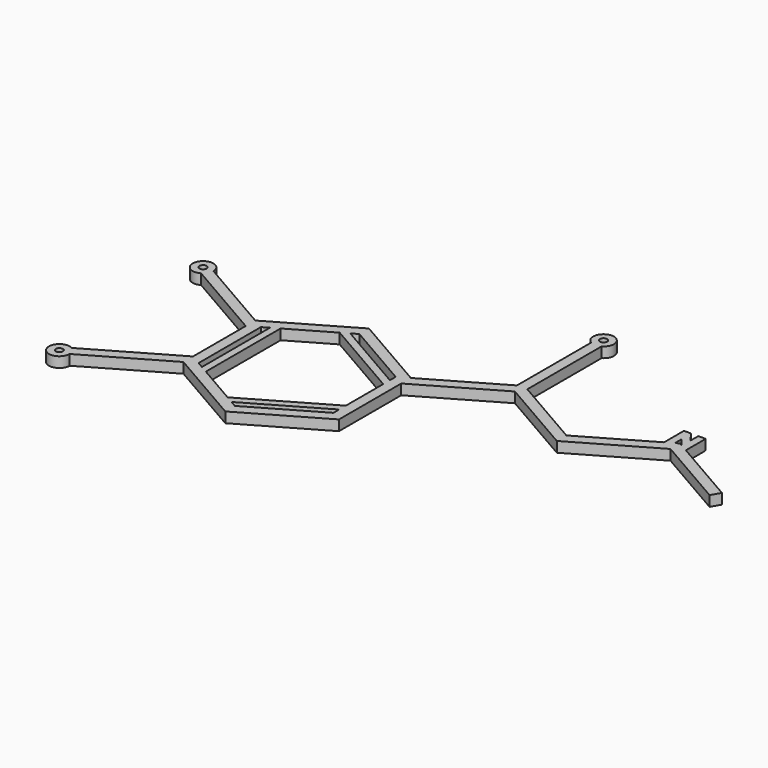
from build123d import *

# Parameters (mm, degrees)
F0_R     = 0.4318
F0_R_2   = 0.4445
F1_DEPTH = 1.27
F3_DEPTH = 1.27


# Not quite as in the source:
# - ends of sketch curves that miss each other by under 0.0002 mm in the source are joined


with BuildPart() as f1:
    # F0 (on Top) → F1 (new body)
    with BuildSketch(Plane.XY):
        with BuildLine():
            Line((9.5249989071, 5.499263207), (-2.1858e-06, 10.9985226281))
            Line((-2.1858e-06, 10.9985226281), (-9.5250010929, 5.499259421))
            Line((-9.5250010929, 5.499259421), (-19.0459112442, 10.9961569369))
            ThreePointArc((-19.0459112442, 10.9961569369), (-21.4157534444, 11.6311591353), (-19.6809068475, 9.8963021357))
            Line((-19.6809068475, 9.8963021357), (-9.5250008015, 4.0327897373))
            Line((-9.5250008015, 4.0327897373), (-9.5249991985, -4.0327941963))
            Line((-9.5249991985, -4.0327941963), (-19.6850080876, -9.8986699867))
            ThreePointArc((-19.6850080876, -9.8986699867), (-21.4198613847, -11.6335212151), (-19.0500087433, -10.9985226281))
            Line((-19.0500087433, -10.9985226281), (-9.5249989071, -5.499263207))
            Line((-9.5249989071, -5.499263207), (2.1858e-06, -10.9985226281))
            Line((2.1858e-06, -10.9985226281), (9.5250010929, -5.499259421))
            Line((9.5250010929, -5.499259421), (9.5249991985, 4.0327941963))
            Line((9.5249991985, 4.0327941963), (19.0500087433, 9.5320534491))
            Line((19.0500087433, 9.5320534491), (28.5750185796, 4.0327940281))
            Line((28.5750185796, 4.0327940281), (38.1000284158, 9.5320534491))
            Line((38.1000284158, 9.5320534491), (46.9900389078, 4.3994105656))
            Line((46.9900389078, 4.3994105656), (47.625038252, 5.499263207))
            Line((47.625038252, 5.499263207), (39.3991596309, 10.2484699041))
            Line((39.3991596309, 10.2484699041), (39.3991596309, 10.224751758))
            Line((39.3991596309, 10.224751758), (38.673771624, 10.6672722885))
            Line((38.673771624, 10.6672722885), (38.1000284158, 10.9985226281))
            Line((38.1000284158, 10.9985226281), (37.6488161101, 10.7380154406))
            Line((37.6488161101, 10.7380154406), (37.6488161101, 10.731614756))
            Line((37.6488161101, 10.731614756), (36.7598161101, 10.224751758))
            Line((36.7598161101, 10.224751758), (28.5750185796, 5.499263207))
            Line((28.5750185796, 5.499263207), (19.6850087433, 10.6319053096))
            Line((19.6850087433, 10.6319053096), (19.6850087433, 10.9985226281))
            Line((19.6850087433, 10.9985226281), (19.6850087433, 21.9970528281))
            ThreePointArc((19.6850087433, 21.9970528281), (19.0500083949, 24.3669048897), (18.4150080465, 21.9970528281))
            Line((18.4150080465, 21.9970528281), (18.4150080465, 10.9985226281))
            Line((18.4150080465, 10.9985226281), (18.4150080465, 10.6319053096))
            Line((18.4150080465, 10.6319053096), (9.5249989071, 5.499263207))
        make_face()
        with Locations((-20.3200087433, -10.9985218709)):
            Circle(F0_R, mode=Mode.SUBTRACT)
        Polygon((8.2550007723, -3.8861430213), (8.2550009472, -4.7660248316), (1.8944e-06, -9.5320529443), (-0.761998193, -9.0921121906), align=None, mode=Mode.SUBTRACT)
        Polygon((-8.255, -1.6406e-06), (-8.2550009472, 4.7660248316), (-7.493, 5.2059664855), (-7.493, -1.6406e-06), (-7.493, -5.2059682691), (-8.2549990528, -4.7660281127), align=None, mode=Mode.SUBTRACT)
        Polygon((-6.604, -5.499263207), (-6.604, 5.7192311104), (-1.6510017049, 8.5788473218), (8.2549994317, 2.8596175239), (8.2550005683, -2.8596142427), (-1.6509982951, -8.578847978), (-6.604, -5.7192324228), align=None, mode=Mode.SUBTRACT)
        with Locations((-20.3159024508, 10.9961569369)):
            Circle(F0_R_2, mode=Mode.SUBTRACT)
        Polygon((-1.8944e-06, 9.5320529443), (8.2549990528, 4.7660281127), (8.2549992277, 3.8861463025), (-0.762001807, 9.0921118878), align=None, mode=Mode.SUBTRACT)
        with Locations((19.0500083949, 23.0969048897)):
            Circle(F0_R_2, mode=Mode.SUBTRACT)
        Polygon((36.7598161101, 10.731614756), (36.7598161101, 10.224751758), (37.6488161101, 10.7380154406), (37.6488161101, 11.8624546668), (38.5683002365, 10.731614756), (38.673771624, 10.6672722885), (39.3991596309, 10.2484699041), (39.3991596309, 10.731614756), (39.3991596309, 13.271614756), (38.5101596309, 13.271614756), (38.5101596309, 12.0436610678), (37.6488161101, 13.271614756), (36.7598161101, 13.271614756), align=None)
        Polygon((37.6488161101, 10.7380154406), (36.7598161101, 10.224751758), (37.6488161101, 10.731614756), align=None)
        Polygon((39.3991596309, 10.2484699041), (38.673771624, 10.6672722885), (39.3991596309, 10.224751758), align=None)
    extrude(amount=F1_DEPTH)

    # F2 (on Top) → F3 (join)
    with BuildSketch(Plane.XY):
        Polygon((37.6677321614, 13.1759580532), (36.7787321614, 13.1759580532), (36.7787321614, 10.6359580532), (36.7787321614, 10.1290950552), (37.6677321614, 10.6359580532), (37.6677321614, 11.7667979639), (38.5872162879, 10.6359580532), (39.4180756822, 10.1290950552), (39.4180756822, 10.6359580532), (39.4180756822, 13.1759580532), (38.5290756822, 13.1759580532), (38.5290756822, 11.948004365), align=None)
    extrude(amount=F3_DEPTH)


solid = f1.part
